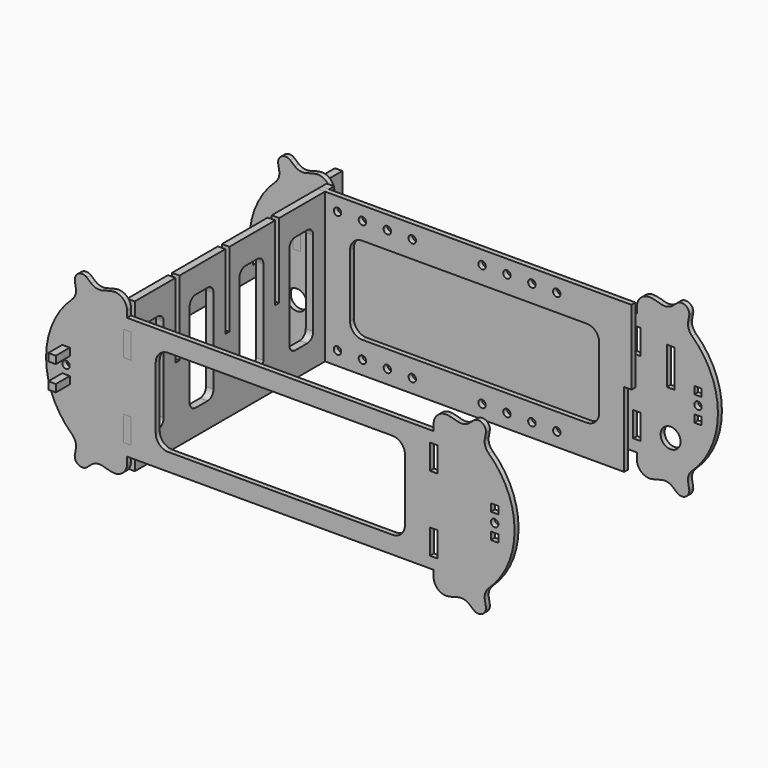
from build123d import *

# Parameters (mm, degrees)
F0_R        = 4
F0_W        = 3
F0_H        = 15
F1_DEPTH    = 2
F2_T1_DEPTH = 2
F2_T3_DEPTH = 31.6693441323
F3_W        = 2
F3_H        = 15
F4_DEPTH    = 3
F5_W        = 3
F5_H        = 10
F6_DEPTH    = 25
F7_W        = 2
F7_H        = 10
F8_DEPTH    = 3
F9_R        = 1.5
F9_W        = 3
F9_H        = 30
F10_DEPTH   = 2
F11_W       = 3
F11_H       = 10
F12_DEPTH   = 2
F13_W       = 3
F13_H       = 3
F13_R       = 1.5
F14_DEPTH   = 123.001
F15_W       = 2
F15_H       = 3
F14_FACE_W  = 2
F14_FACE_H  = 3
F16_DEPTH   = 3
F17_W       = 3
F17_H       = 3
F18_DEPTH   = 7


# Not quite as in the source:
# - a fillet or chamfer that OpenCascade refuses, or shapes differently, is made with other operations: its cross-section is extruded or revolved along the edge and cut away or added
# - ends of sketch curves that miss each other by under 0.0002 mm in the source are joined


with BuildPart() as f1:
    # F0 (on Front) → F1 (new body)
    with BuildSketch(Plane.XZ):
        with BuildLine():
            ThreePointArc((-76.5000003175, 31.1769145362), (-76.7810769564, 32.4447693215), (-77.5716374885, 33.4750478656))
            ThreePointArc((-77.5716374885, 33.4750478656), (-81.0000003175, 33.7749907476), (-82.4544235766, 30.6559700032))
            ThreePointArc((-82.4544235766, 30.6559700032), (-79.2385330893, 28.188330442), (-76.5000003175, 31.1769145362))
        make_face()
        with BuildLine():
            ThreePointArc((82.5000003175, 31.1769145362), (80.7678551027, 33.8958378973), (77.5716374885, 33.4750478656))
            ThreePointArc((77.5716374885, 33.4750478656), (78.0000003175, 28.5788383249), (82.4544235766, 30.6559700032))
            ThreePointArc((82.4544235766, 30.6559700032), (82.4885844118, 30.915447308), (82.5000003175, 31.1769145362))
        make_face()
        with BuildLine():
            ThreePointArc((82.5000003175, -31.1769145362), (82.4885844118, -30.915447308), (82.4544235766, -30.6559700032))
            ThreePointArc((82.4544235766, -30.6559700032), (78.0000003175, -28.5788383249), (77.5716374885, -33.4750478656))
            ThreePointArc((77.5716374885, -33.4750478656), (80.7678551027, -33.8958378973), (82.5000003175, -31.1769145362))
        make_face()
        with BuildLine():
            ThreePointArc((-76.5000003175, -31.1769145362), (-79.2385330893, -28.188330442), (-82.4544235766, -30.6559700032))
            ThreePointArc((-82.4544235766, -30.6559700032), (-81.0000003175, -33.7749907476), (-77.5716374885, -33.4750478656))
            ThreePointArc((-77.5716374885, -33.4750478656), (-76.7810769564, -32.4447693215), (-76.5000003175, -31.1769145362))
        make_face()
        with BuildLine():
            ThreePointArc((-81.5579830015, 25.5720028674), (-77.7500003175, 28.145825623), (-73.6170130844, 30.1567239867))
            Line((-73.6170130844, 30.1567239867), (-77.5716374885, 33.4750478656))
            ThreePointArc((-77.5716374885, 33.4750478656), (-76.7810769564, 32.4447693215), (-76.5000003175, 31.1769145362))
            ThreePointArc((-76.5000003175, 31.1769145362), (-79.2385330893, 28.188330442), (-82.4544235766, 30.6559700032))
            Line((-82.4544235766, 30.6559700032), (-81.5579830015, 25.5720028674))
        make_face()
        with BuildLine():
            ThreePointArc((-73.6170130844, -30.1567239867), (-77.7500003175, -28.145825623), (-81.5579830015, -25.5720028674))
            Line((-81.5579830015, -25.5720028674), (-82.4544235766, -30.6559700032))
            ThreePointArc((-82.4544235766, -30.6559700032), (-79.2385330893, -28.188330442), (-76.5000003175, -31.1769145362))
            ThreePointArc((-76.5000003175, -31.1769145362), (-76.7810769564, -32.4447693215), (-77.5716374885, -33.4750478656))
            Line((-77.5716374885, -33.4750478656), (-73.6170130844, -30.1567239867))
        make_face()
        with BuildLine():
            Line((82.4544235766, -30.6559700032), (81.5579830015, -25.5720028674))
            ThreePointArc((81.5579830015, -25.5720028674), (77.750000154, -28.1458253508), (73.6170129961, -30.156723767))
            Line((73.6170129961, -30.156723767), (77.5716374885, -33.4750478656))
            ThreePointArc((77.5716374885, -33.4750478656), (78.0000003175, -28.5788383249), (82.4544235766, -30.6559700032))
        make_face()
        with BuildLine():
            Line((77.5716374885, 33.4750478656), (73.6170130844, 30.1567239867))
            ThreePointArc((73.6170130844, 30.1567239867), (77.750000154, 28.1458253508), (81.5579827596, 25.572002559))
            Line((81.5579827596, 25.572002559), (82.4544235766, 30.6559700032))
            ThreePointArc((82.4544235766, 30.6559700032), (78.0000003175, 28.5788383249), (77.5716374885, 33.4750478656))
        make_face()
        with BuildLine():
            Line((-61.5000003175, 24.5), (-61.5000003175, 32.5))
            ThreePointArc((-61.5000003175, 32.5), (-67.6707567717, 31.9088038758), (-73.6170130844, 30.1567239867))
            ThreePointArc((-73.6170130844, 30.1567239867), (-77.7500003175, 28.145825623), (-81.5579830015, 25.5720028674))
            ThreePointArc((-81.5579830015, 25.5720028674), (-94.0000003175, 0), (-81.5579830015, -25.5720028674))
            ThreePointArc((-81.5579830015, -25.5720028674), (-77.7500003175, -28.145825623), (-73.6170130844, -30.1567239867))
            ThreePointArc((-73.6170130844, -30.1567239867), (-67.6707567717, -31.9088038758), (-61.5000003175, -32.5))
            Line((-61.5000003175, -32.5), (-61.5000003175, -24.5))
            Line((-61.5000003175, -24.5), (61.4999996825, -24.5))
            Line((61.4999996825, -24.5), (61.4999996825, -32.5))
            ThreePointArc((61.4999996825, -32.5), (67.6707564259, -31.9088038198), (73.6170129961, -30.156723767))
            ThreePointArc((73.6170129961, -30.156723767), (77.750000154, -28.1458253508), (81.5579827596, -25.572002559))
            ThreePointArc((81.5579827596, -25.572002559), (93.9999996825, 0), (81.5579827596, 25.572002559))
            ThreePointArc((81.5579827596, 25.572002559), (77.750000154, 28.1458253508), (73.6170129961, 30.156723767))
            ThreePointArc((73.6170129961, 30.156723767), (67.6707564259, 31.9088038198), (61.4999996825, 32.5))
            Line((61.4999996825, 32.5), (61.4999996825, 24.5))
            Line((61.4999996825, 24.5), (-61.5000003175, 24.5))
        make_face()
        with Locations((-75, -15)):
            Circle(F0_R, mode=Mode.SUBTRACT)
        with Locations((75, -15)):
            Circle(F0_R, mode=Mode.SUBTRACT)
        with Locations((-75, 10)):
            Rectangle(F0_W, F0_H, mode=Mode.SUBTRACT)
        with Locations((75, 10)):
            Rectangle(F0_W, F0_H, mode=Mode.SUBTRACT)
    extrude(amount=F1_DEPTH)

    # F2: fillet of radius 5 on 12 edges, made by hand

    # F2_s2 → F2_t1 (join)
    with BuildSketch(Plane.XZ):
        with BuildLine():
            ThreePointArc((-71.1118245729, 31.046140412), (-73.5787498539, 30.921092942), (-75.8045048145, 31.9922474906))
            Line((-75.8045048145, 31.9922474906), (-73.6170130844, 30.1567239867))
            ThreePointArc((-73.6170130844, 30.1567239867), (-72.3735165372, 30.6270574006), (-71.1118245729, 31.046140412))
        make_face()
        with BuildLine():
            ThreePointArc((-82.0538471201, 28.3841880282), (-82.2390775499, 25.9210504154), (-83.5808344761, 23.8471541879))
            ThreePointArc((-83.5808344761, 23.8471541879), (-82.5870519598, 24.730269975), (-81.5579830015, 25.5720028674))
            Line((-81.5579830015, 25.5720028674), (-82.0538471201, 28.3841880282))
        make_face()
        with BuildLine():
            ThreePointArc((75.8045046433, 31.992247347), (73.578749651, 30.9210927919), (71.1118243399, 31.0461402876))
            ThreePointArc((71.1118243399, 31.0461402876), (72.3735163804, 30.6270572308), (73.6170130402, 30.1567238768))
            Line((73.6170130402, 30.1567238768), (75.8045046433, 31.992247347))
        make_face()
        with BuildLine():
            ThreePointArc((83.5808342518, 23.8471538076), (82.2390773465, 25.9210501022), (82.05384699, 28.3841877655))
            Line((82.05384699, 28.3841877655), (81.5579827596, 25.572002559))
            ThreePointArc((81.5579827596, 25.572002559), (82.5870517278, 24.7302696313), (83.5808342518, 23.8471538076))
        make_face()
        with BuildLine():
            ThreePointArc((82.0538470309, -28.3841875227), (82.2390774449, -25.9210499569), (83.5808343142, -23.8471537498))
            ThreePointArc((83.5808343142, -23.8471537498), (82.5870517571, -24.7302696063), (81.5579828805, -25.5720027132))
            Line((81.5579828805, -25.5720027132), (82.0538470309, -28.3841875227))
        make_face()
        with BuildLine():
            ThreePointArc((71.111824389, -31.0461402724), (73.5787497567, -30.9210927843), (75.8045047827, -31.9922473989))
            Line((75.8045047827, -31.9922473989), (73.6170129961, -30.156723767))
            ThreePointArc((73.6170129961, -30.156723767), (72.3735164023, -30.627057223), (71.111824389, -31.0461402724))
        make_face()
        with BuildLine():
            ThreePointArc((-75.8045048145, -31.9922474906), (-73.5787498539, -30.921092942), (-71.1118245729, -31.046140412))
            ThreePointArc((-71.1118245729, -31.046140412), (-72.3735165372, -30.6270574006), (-73.6170130844, -30.1567239867))
            Line((-73.6170130844, -30.1567239867), (-75.8045048145, -31.9922474906))
        make_face()
        with BuildLine():
            ThreePointArc((-83.5808344761, -23.8471541879), (-82.2390775499, -25.9210504154), (-82.0538471201, -28.3841880282))
            Line((-82.0538471201, -28.3841880282), (-81.5579830015, -25.5720028674))
            ThreePointArc((-81.5579830015, -25.5720028674), (-82.5870519598, -24.730269975), (-83.5808344761, -23.8471541879))
        make_face()
    extrude(amount=F2_T1_DEPTH)

    # F2_s4 → F2_t3 (cut)
    with BuildSketch(Plane.XZ.offset(-14.8346720662)):
        with BuildLine():
            ThreePointArc((-61.5000003175, 27.041634566), (-63.3019895722, 30.8851651399), (-67.4090912266, 31.9582953962))
            ThreePointArc((-67.4090912266, 31.9582953962), (-64.4669347308, 32.3642905096), (-61.5000003175, 32.5))
            Line((-61.5000003175, 32.5), (-61.5000003175, 27.041634566))
        make_face()
        with BuildLine():
            ThreePointArc((67.4090905916, 31.9582953962), (63.3019889371, 30.8851651399), (61.4999996825, 27.041634566))
            Line((61.4999996825, 27.041634566), (61.4999996825, 32.5))
            ThreePointArc((61.4999996825, 32.5), (64.4669340957, 32.3642905096), (67.4090905916, 31.9582953962))
        make_face()
        with BuildLine():
            ThreePointArc((61.4999996825, -27.041634566), (63.3019889371, -30.8851651399), (67.4090905916, -31.9582953962))
            ThreePointArc((67.4090905916, -31.9582953962), (64.4669340957, -32.3642905096), (61.4999996825, -32.5))
            Line((61.4999996825, -32.5), (61.4999996825, -27.041634566))
        make_face()
        with BuildLine():
            ThreePointArc((-67.4090912266, -31.9582953962), (-63.3019895722, -30.8851651399), (-61.5000003175, -27.041634566))
            Line((-61.5000003175, -27.041634566), (-61.5000003175, -32.5))
            ThreePointArc((-61.5000003175, -32.5), (-64.4669347308, -32.3642905096), (-67.4090912266, -31.9582953962))
        make_face()
    extrude(amount=F2_T3_DEPTH, mode=Mode.SUBTRACT)

    # F5 (on face) → F6 (cut)
    with BuildSketch(Plane.XZ.offset(2)):
        with Locations((61.5, 15)):
            Rectangle(F5_W, F5_H)
        with Locations((61.5, -15)):
            Rectangle(F5_W, F5_H)
        with Locations((-61.5, 15)):
            Rectangle(F5_W, F5_H)
        with Locations((-61.5, -15)):
            Rectangle(F5_W, F5_H)
    extrude(amount=-F6_DEPTH, mode=Mode.SUBTRACT)


with BuildPart() as f4:
    # F3 (on face) → F4 (new body)
    with BuildSketch(Plane(origin=(-73.5, 0, 0), x_dir=(0, -1, 0), z_dir=(-1, 0, 0))):
        with Locations((1, 10)):
            Rectangle(F3_W, F3_H)
        Polygon((0, 2.5), (0, 17.5), (0, 22.5), (-19, 22.5), (-19, -2.5), (0, -2.5), align=None)
    extrude(amount=F4_DEPTH)


with BuildPart() as f8:
    # F7 (on face) → F8 (new body)
    with BuildSketch(Plane.YZ.offset(-63)):
        Polygon((-2, 20), (-2, 30), (-4.5775633082, 30), (-4.5775633082, 0), (-6.5775633082, 0), (-6.5775633082, 30), (-29.5775633082, 30), (-29.5775633082, 0), (-31.5775633082, 0), (-31.5775633082, 30), (-54.5775633082, 30), (-54.5775633082, 0), (-56.5775633082, 0), (-56.5775633082, 30), (-79.5775633082, 30), (-79.5775633082, 0), (-81.5775633082, 0), (-81.5775633082, 30), (-102, 30), (-102, 20), (-102, 10), (-102, -10), (-102, -20), (-102, -30), (-2, -30), (-2, -20), (-2, -10), (-2, 10), align=None)
        with BuildLine():
            Line((-96.5, 20), (-90.5, 20))
            ThreePointArc((-90.5, 20), (-88.3786796564, 19.1213203436), (-87.5, 17))
            Line((-87.5, 17), (-87.5, -17))
            ThreePointArc((-87.5, -17), (-88.3786796564, -19.1213203436), (-90.5, -20))
            Line((-90.5, -20), (-96.5, -20))
            ThreePointArc((-96.5, -20), (-98.6213203436, -19.1213203436), (-99.5, -17))
            Line((-99.5, -17), (-99.5, 17))
            ThreePointArc((-99.5, 17), (-98.6213203436, 19.1213203436), (-96.5, 20))
        make_face(mode=Mode.SUBTRACT)
        with BuildLine():
            Line((-71.5, 20), (-65.5, 20))
            ThreePointArc((-65.5, 20), (-63.3786796564, 19.1213203436), (-62.5, 17))
            Line((-62.5, 17), (-62.5, -17))
            ThreePointArc((-62.5, -17), (-63.3786796564, -19.1213203436), (-65.5, -20))
            Line((-65.5, -20), (-71.5, -20))
            ThreePointArc((-71.5, -20), (-73.6213203436, -19.1213203436), (-74.5, -17))
            Line((-74.5, -17), (-74.5, 17))
            ThreePointArc((-74.5, 17), (-73.6213203436, 19.1213203436), (-71.5, 20))
        make_face(mode=Mode.SUBTRACT)
        with BuildLine():
            Line((-46.5, 20), (-40.5, 20))
            ThreePointArc((-40.5, 20), (-38.3786796564, 19.1213203436), (-37.5, 17))
            Line((-37.5, 17), (-37.5, -17))
            ThreePointArc((-37.5, -17), (-38.3786796564, -19.1213203436), (-40.5, -20))
            Line((-40.5, -20), (-46.5, -20))
            ThreePointArc((-46.5, -20), (-48.6213203436, -19.1213203436), (-49.5, -17))
            Line((-49.5, -17), (-49.5, 17))
            ThreePointArc((-49.5, 17), (-48.6213203436, 19.1213203436), (-46.5, 20))
        make_face(mode=Mode.SUBTRACT)
        with BuildLine():
            Line((-21.5, 20), (-15.5, 20))
            ThreePointArc((-15.5, 20), (-13.3786796564, 19.1213203436), (-12.5, 17))
            Line((-12.5, 17), (-12.5, -17))
            ThreePointArc((-12.5, -17), (-13.3786796564, -19.1213203436), (-15.5, -20))
            Line((-15.5, -20), (-21.5, -20))
            ThreePointArc((-21.5, -20), (-23.6213203436, -19.1213203436), (-24.5, -17))
            Line((-24.5, -17), (-24.5, 17))
            ThreePointArc((-24.5, 17), (-23.6213203436, 19.1213203436), (-21.5, 20))
        make_face(mode=Mode.SUBTRACT)
        with Locations((-103, 15)):
            Rectangle(F7_W, F7_H)
        with Locations((-103, -15)):
            Rectangle(F7_W, F7_H)
        with Locations((-1, 15)):
            Rectangle(F7_W, F7_H)
        with Locations((-1, -15)):
            Rectangle(F7_W, F7_H)
    extrude(amount=F8_DEPTH)


with BuildPart() as f10:
    # F9 (on face) → F10 (new body)
    with BuildSketch(Plane.XZ.offset(4.5775633082)):
        Polygon((60, 30), (-60, 30), (-60, 0), (-60, -30), (60, -30), (60, 0), align=None)
        with Locations((-55, -24.5)):
            Circle(F9_R, mode=Mode.SUBTRACT)
        with Locations((-45, -24.5)):
            Circle(F9_R, mode=Mode.SUBTRACT)
        with Locations((-35, -24.5)):
            Circle(F9_R, mode=Mode.SUBTRACT)
        with Locations((-25, -24.5)):
            Circle(F9_R, mode=Mode.SUBTRACT)
        with Locations((3, -24.5)):
            Circle(F9_R, mode=Mode.SUBTRACT)
        with Locations((13, -24.5)):
            Circle(F9_R, mode=Mode.SUBTRACT)
        with Locations((23, -24.5)):
            Circle(F9_R, mode=Mode.SUBTRACT)
        with Locations((33, -24.5)):
            Circle(F9_R, mode=Mode.SUBTRACT)
        with Locations((-55, 24.5)):
            Circle(F9_R, mode=Mode.SUBTRACT)
        with Locations((-45, 24.5)):
            Circle(F9_R, mode=Mode.SUBTRACT)
        with Locations((-35, 24.5)):
            Circle(F9_R, mode=Mode.SUBTRACT)
        with Locations((-25, 24.5)):
            Circle(F9_R, mode=Mode.SUBTRACT)
        with BuildLine():
            ThreePointArc((-50, 12.5), (-48.5355339059, 16.0355339059), (-45, 17.5))
            Line((-45, 17.5), (45, 17.5))
            ThreePointArc((45, 17.5), (48.5355339059, 16.0355339059), (50, 12.5))
            Line((50, 12.5), (50, -12.5))
            ThreePointArc((50, -12.5), (48.5355339059, -16.0355339059), (45, -17.5))
            Line((45, -17.5), (-45, -17.5))
            ThreePointArc((-45, -17.5), (-48.5355339059, -16.0355339059), (-50, -12.5))
            Line((-50, -12.5), (-50, 12.5))
        make_face(mode=Mode.SUBTRACT)
        with Locations((3, 24.5)):
            Circle(F9_R, mode=Mode.SUBTRACT)
        with Locations((13, 24.5)):
            Circle(F9_R, mode=Mode.SUBTRACT)
        with Locations((23, 24.5)):
            Circle(F9_R, mode=Mode.SUBTRACT)
        with Locations((33, 24.5)):
            Circle(F9_R, mode=Mode.SUBTRACT)
        with Locations((-61.5, 15)):
            Rectangle(F9_W, F9_H)
        with Locations((61.5, 15)):
            Rectangle(F9_W, F9_H)
    extrude(amount=F10_DEPTH)


with BuildPart() as f12:
    # F11 (on face) → F12 (new body)
    with BuildSketch(Plane.XZ.offset(102)):
        with BuildLine():
            Line((61.4999996825, 24.5), (-61.5000003175, 24.5))
            Line((-61.5000003175, 24.5), (-61.5000003175, 27.041634566))
            ThreePointArc((-61.5000003175, 27.041634566), (-63.3019895722, 30.8851651399), (-67.4090912266, 31.9582953962))
            ThreePointArc((-67.4090912266, 31.9582953962), (-69.2738480498, 31.5565728722), (-71.1118245729, 31.046140412))
            ThreePointArc((-71.1118245729, 31.046140412), (-73.5787498539, 30.921092942), (-75.8045048145, 31.9922474906))
            Line((-75.8045048145, 31.9922474906), (-77.5716374885, 33.4750478656))
            ThreePointArc((-77.5716374885, 33.4750478656), (-81.0000003175, 33.7749907476), (-82.4544235766, 30.6559700032))
            Line((-82.4544235766, 30.6559700032), (-82.0538471201, 28.3841880282))
            ThreePointArc((-82.0538471201, 28.3841880282), (-82.2390775499, 25.9210504154), (-83.5808344761, 23.8471541879))
            ThreePointArc((-83.5808344761, 23.8471541879), (-94.0000003175, 0), (-83.5808344761, -23.8471541879))
            ThreePointArc((-83.5808344761, -23.8471541879), (-82.2390775499, -25.9210504154), (-82.0538471201, -28.3841880282))
            Line((-82.0538471201, -28.3841880282), (-82.4544235766, -30.6559700032))
            ThreePointArc((-82.4544235766, -30.6559700032), (-81.0000003175, -33.7749907476), (-77.5716374885, -33.4750478656))
            Line((-77.5716374885, -33.4750478656), (-75.8045048145, -31.9922474906))
            ThreePointArc((-75.8045048145, -31.9922474906), (-73.5787498539, -30.921092942), (-71.1118245729, -31.046140412))
            ThreePointArc((-71.1118245729, -31.046140412), (-69.2738480498, -31.5565728722), (-67.4090912266, -31.9582953962))
            ThreePointArc((-67.4090912266, -31.9582953962), (-63.3019895722, -30.8851651399), (-61.5000003175, -27.041634566))
            Line((-61.5000003175, -27.041634566), (-61.5000003175, -24.5))
            Line((-61.5000003175, -24.5), (61.4999996825, -24.5))
            Line((61.4999996825, -24.5), (61.4999996825, -27.041634566))
            ThreePointArc((61.4999996825, -27.041634566), (63.3019889371, -30.8851651399), (67.4090905916, -31.9582953962))
            ThreePointArc((67.4090905916, -31.9582953962), (69.2738476191, -31.5565728218), (71.1118243399, -31.0461402876))
            ThreePointArc((71.1118243399, -31.0461402876), (73.578749651, -30.9210927919), (75.8045046433, -31.992247347))
            Line((75.8045046433, -31.992247347), (77.5716374885, -33.4750478656))
            ThreePointArc((77.5716374885, -33.4750478656), (81.0000003175, -33.7749907476), (82.4544235766, -30.6559700032))
            Line((82.4544235766, -30.6559700032), (82.0538470309, -28.3841875227))
            ThreePointArc((82.0538470309, -28.3841875227), (82.2390774449, -25.9210499569), (83.5808343142, -23.8471537498))
            ThreePointArc((83.5808343142, -23.8471537498), (93.9999996825, 0), (83.5808343142, 23.8471537498))
            ThreePointArc((83.5808343142, 23.8471537498), (82.2390774449, 25.9210499569), (82.0538470309, 28.3841875227))
            Line((82.0538470309, 28.3841875227), (82.4544235766, 30.6559700032))
            ThreePointArc((82.4544235766, 30.6559700032), (81.0000003175, 33.7749907476), (77.5716374885, 33.4750478656))
            Line((77.5716374885, 33.4750478656), (75.8045046433, 31.992247347))
            ThreePointArc((75.8045046433, 31.992247347), (73.578749651, 30.9210927919), (71.1118243399, 31.0461402876))
            ThreePointArc((71.1118243399, 31.0461402876), (69.2738476191, 31.5565728218), (67.4090905916, 31.9582953962))
            ThreePointArc((67.4090905916, 31.9582953962), (63.3019889371, 30.8851651399), (61.4999996825, 27.041634566))
            Line((61.4999996825, 27.041634566), (61.4999996825, 24.5))
        make_face()
        with Locations((-61.5, -15)):
            Rectangle(F11_W, F11_H, mode=Mode.SUBTRACT)
        with Locations((61.5, -15)):
            Rectangle(F11_W, F11_H, mode=Mode.SUBTRACT)
        with Locations((-61.5, 15)):
            Rectangle(F11_W, F11_H, mode=Mode.SUBTRACT)
        with BuildLine():
            ThreePointArc((-50, 12.5), (-48.5355339059, 16.0355339059), (-45, 17.5))
            Line((-45, 17.5), (0, 17.5))
            Line((0, 17.5), (45, 17.5))
            ThreePointArc((45, 17.5), (48.5355339059, 16.0355339059), (50, 12.5))
            Line((50, 12.5), (50, -12.5))
            ThreePointArc((50, -12.5), (48.5355339059, -16.0355339059), (45, -17.5))
            Line((45, -17.5), (-45, -17.5))
            ThreePointArc((-45, -17.5), (-48.5355339059, -16.0355339059), (-50, -12.5))
            Line((-50, -12.5), (-50, 12.5))
        make_face(mode=Mode.SUBTRACT)
        with Locations((61.5, 15)):
            Rectangle(F11_W, F11_H, mode=Mode.SUBTRACT)
    extrude(amount=F12_DEPTH)


with BuildPart() as f14_tool:
    # F13 (on face) → F14 (new body, through all)
    with BuildSketch(Plane.XZ.offset(104)):
        with Locations((-86, 5)):
            Rectangle(F13_W, F13_H)
        with Locations((86, 5)):
            Rectangle(F13_W, F13_H)
        with Locations((-86, -5)):
            Rectangle(F13_W, F13_H)
        with Locations((86, -5)):
            Rectangle(F13_W, F13_H)
        with Locations((-86, 0)):
            Circle(F13_R)
        with Locations((86, 0)):
            Circle(F13_R)
    extrude(amount=-F14_DEPTH)


with BuildPart() as f1_1:
    add(f1.part)

    # F14: cut by f14_tool
    add(f14_tool.part, mode=Mode.SUBTRACT)


with BuildPart() as f12_1:
    add(f12.part)

    # F14: cut by f14_tool
    add(f14_tool.part, mode=Mode.SUBTRACT)


with BuildPart() as f16:
    # F15 (on face) + F14_face (on face) → F16 (new body)
    with BuildSketch(Plane(origin=(-84.5, 0, 0), x_dir=(0, -1, 0), z_dir=(-1, 0, 0))):
        Polygon((102, 6.5), (2, 6.5), (2, 1.65), (4, 1.65), (4, 3.5), (7, 3.5), (7, 1.65), (12, 1.65), (12, -1.65), (7, -1.65), (7, -3.5), (4, -3.5), (4, -1.65), (2, -1.65), (2, -6.5), (102, -6.5), (102, -1.65), (100, -1.65), (100, -3.5), (97, -3.5), (97, -1.65), (92, -1.65), (92, 1.65), (97, 1.65), (97, 3.5), (100, 3.5), (100, 1.65), (102, 1.65), (102, 3.5), align=None)
        with Locations((103, 5)):
            Rectangle(F15_W, F15_H)
    with BuildSketch(Plane(origin=(-84.5, -103, 5), x_dir=(0, -1, 0), z_dir=(-1, 0, 0))):
        with Locations((-102, 0)):
            Rectangle(F14_FACE_W, F14_FACE_H)
        with Locations((-102, -10)):
            Rectangle(F14_FACE_W, F14_FACE_H)
        with Locations((0, -10)):
            Rectangle(F14_FACE_W, F14_FACE_H)
    extrude(amount=F16_DEPTH)

    # F17 (on face) → F18 (join)
    with BuildSketch(Plane.XZ.offset(104)):
        with Locations((-86, -5)):
            Rectangle(F17_W, F17_H)
        with Locations((-86, 5)):
            Rectangle(F17_W, F17_H)
    extrude(amount=F18_DEPTH)


solid = Compound([f4.part, f8.part, f10.part, f1_1.part, f12_1.part, f16.part])
